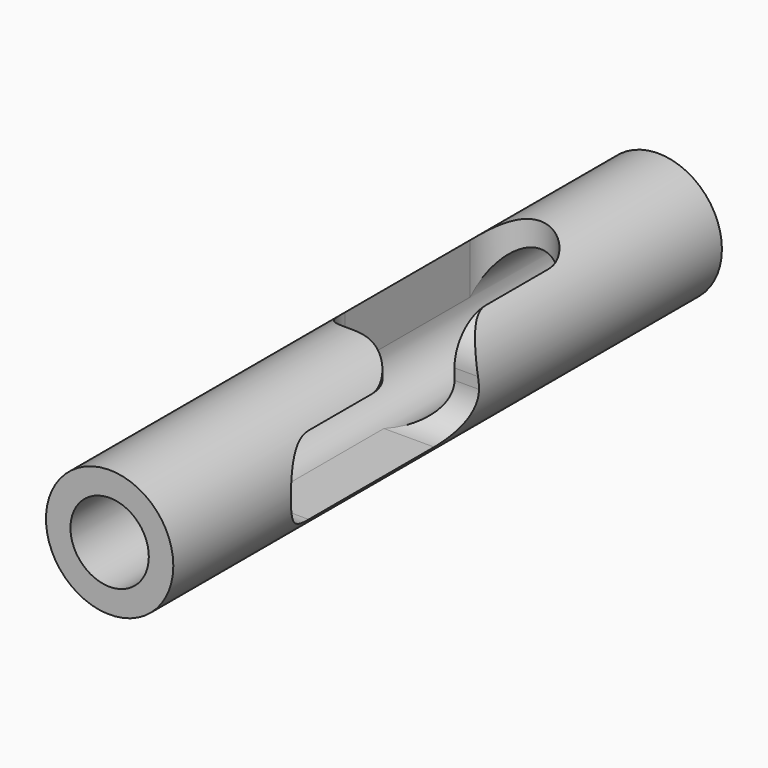
from build123d import *

# Parameters (mm, degrees)
F0_R         = 65
F0_R_2       = 40
F1_DEPTH     = 350
F3_DEPTH     = 65.001
F5_DEPTH     = 65.0010001
F6_T4_DEPTH  = 251.2347538298
F6_S5_R      = 65
F6_T6_DEPTH  = 130
F6_S7_R      = 40
F6_T8_DEPTH  = 130
F6_T12_DEPTH = 251.2347538298
F6_S13_R     = 65
F6_T14_DEPTH = 130
F6_S15_R     = 40
F6_T16_DEPTH = 130
F8_DEPTH     = 65.0010001
F10_DEPTH    = 65.0010001


# Not quite as in the source:
# - a fillet or chamfer that OpenCascade refuses, or shapes differently, is made with other operations: its cross-section is extruded or revolved along the edge and cut away or added


with BuildPart() as f1:
    # F0 (on Front) → F1 (new body, symmetric)
    with BuildSketch(Plane.XZ):
        Circle(F0_R)
        Circle(F0_R_2, mode=Mode.SUBTRACT)
    extrude(amount=F1_DEPTH, both=True)

    # F2 (on Top) → F3 (cut, through all)
    with BuildSketch(Plane.XY):
        with BuildLine():
            ThreePointArc((-40, 160), (0, 120), (40, 160))
            ThreePointArc((40, 160), (0, 200), (-40, 160))
        make_face()
        with BuildLine():
            Line((40, 40), (40, 160))
            ThreePointArc((40, 160), (0, 120), (-40, 160))
            Line((-40, 160), (-40, -40))
            Line((-40, -40), (65, -40))
            Line((65, -40), (65, 40))
            Line((65, 40), (40, 40))
        make_face()
    extrude(amount=F3_DEPTH, mode=Mode.SUBTRACT)

    # F4 (on Right) → F5 (cut, through all)
    with BuildSketch(Plane.YZ):
        with BuildLine():
            ThreePointArc((-160, -40), (-131.7157287525, -28.2842712475), (-120, 0))
            ThreePointArc((-120, 0), (-131.7157287525, 28.2842712475), (-160, 40))
            ThreePointArc((-160, 40), (-200, 0), (-160, -40))
        make_face()
        with BuildLine():
            ThreePointArc((-160, 40), (-131.7157287525, 28.2842712475), (-120, 0))
            ThreePointArc((-120, 0), (-131.7157287525, -28.2842712475), (-160, -40))
            Line((-160, -40), (40, -40))
            Line((40, -40), (40, 65))
            Line((40, 65), (-40, 65))
            Line((-40, 65), (-40, 40))
            Line((-40, 40), (-160, 40))
        make_face()
    extrude(amount=F5_DEPTH, mode=Mode.SUBTRACT)

    # F6: fillet of radius 40 on 2 edges, made by hand


with BuildPart() as f6_tool2:
    # F6_s3 → F6_t4 (new body)
    with BuildSketch(Plane.YZ.offset(-100)):
        with BuildLine():
            ThreePointArc((0, -40), (28.2842712475, -28.2842712475), (40, 0))
            Line((40, 0), (40, -40))
            Line((40, -40), (0, -40))
        make_face()
    extrude(amount=F6_T4_DEPTH)

    # F6_s5 → F6_t6 (intersect, symmetric)
    with BuildSketch(Plane.XZ.offset(-20)):
        Circle(F6_S5_R)
    extrude(amount=F6_T6_DEPTH, both=True, mode=Mode.INTERSECT)

    # F6_s7 → F6_t8 (cut, symmetric)
    with BuildSketch(Plane.XZ.offset(-20)):
        Circle(F6_S7_R)
    extrude(amount=F6_T8_DEPTH, both=True, mode=Mode.SUBTRACT)


with BuildPart() as f1_1:
    add(f1.part)

    # F6_t1: union F6_tool2
    add(f6_tool2.part)


with BuildPart() as f6_tool10:
    # F6_s11 → F6_t12 (new body)
    with BuildSketch(Plane.XY.offset(-100)):
        with BuildLine():
            ThreePointArc((-40, 0), (-28.2842712475, -28.2842712475), (0, -40))
            Line((0, -40), (-40, -40))
            Line((-40, -40), (-40, 0))
        make_face()
    extrude(amount=F6_T12_DEPTH)

    # F6_s13 → F6_t14 (intersect, symmetric)
    with BuildSketch(Plane.XZ.offset(20)):
        Circle(F6_S13_R)
    extrude(amount=F6_T14_DEPTH, both=True, mode=Mode.INTERSECT)

    # F6_s15 → F6_t16 (cut, symmetric)
    with BuildSketch(Plane.XZ.offset(20)):
        Circle(F6_S15_R)
    extrude(amount=F6_T16_DEPTH, both=True, mode=Mode.SUBTRACT)


with BuildPart() as f1_2:
    add(f1_1.part)

    # F6_t9: union F6_tool10
    add(f6_tool10.part)

    # F7 (on Top) → F8 (cut, through all)
    with BuildSketch(Plane.XY):
        with BuildLine():
            ThreePointArc((11.2347538298, -40), (39.5190250773, -51.7157287525), (51.2347538298, -80))
            Line((51.2347538298, -80), (51.2347538298, -40))
            Line((51.2347538298, -40), (11.2347538298, -40))
        make_face()
    extrude(amount=F8_DEPTH, mode=Mode.SUBTRACT)

    # F9 (on Right) → F10 (cut, through all)
    with BuildSketch(Plane.YZ):
        with BuildLine():
            ThreePointArc((40, 11.2347538298), (51.7157287525, 39.5190250773), (80, 51.2347538298))
            Line((80, 51.2347538298), (40, 51.2347538298))
            Line((40, 51.2347538298), (40, 11.2347538298))
        make_face()
    extrude(amount=F10_DEPTH, mode=Mode.SUBTRACT)


solid = f1_2.part
